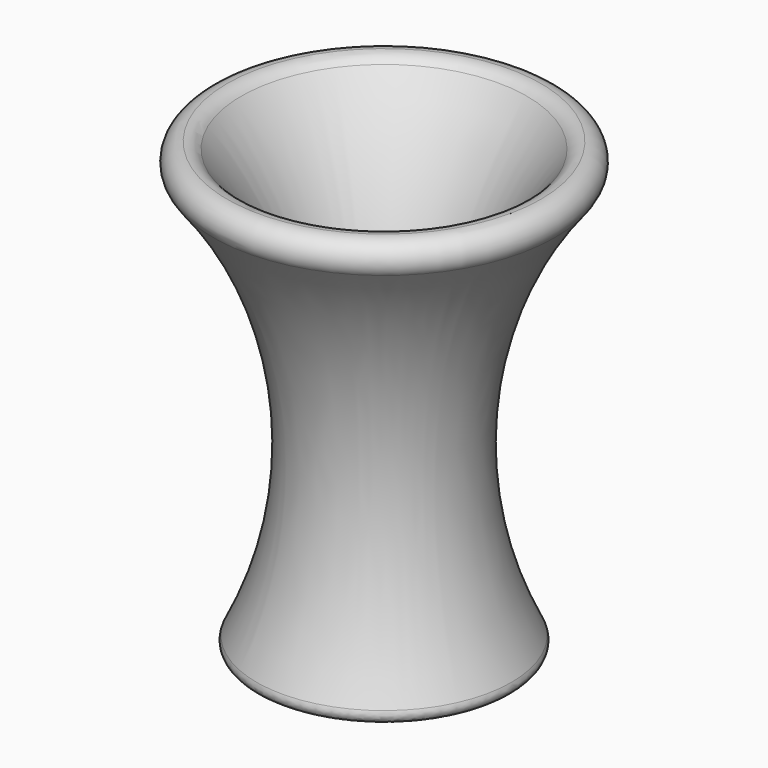
from build123d import *

# Parameters (mm, degrees)
F2_T = -5.08
F4_R = 2.54
F5_R = 1.27


# Not quite as in the source:
# - a fillet or chamfer that OpenCascade refuses, or shapes differently, is made with other operations: its cross-section is extruded or revolved along the edge and cut away or added


with BuildPart() as f1:
    # F0 (on Front) → F1 (revolve)
    with BuildSketch(Plane.XZ):
        with BuildLine():
            Line((67.6932582283, 49.1091830879), (39.7532582283, 49.1091830879))
            Line((39.7532582283, 49.1091830879), (39.7532582283, -14.3908169121))
            Line((39.7532582283, -14.3908169121), (58.8032582283, -14.3908169121))
            ThreePointArc((58.8032582283, -14.3908169121), (52.6399701012, 18.8443434257), (67.6932582283, 49.1091830879))
        make_face()
    revolve(axis=Axis((39.7532582283, 0, 17.3591830879), (0, 0, -1)))

    # F2
    f2_openings = [f1.faces().sort_by_distance(p)[0] for p in [
        (39.753258, 0, 49.109183),
    ]]
    offset(amount=F2_T, openings=f2_openings)

    # F3: fillet of radius 2.54 on 2 edges, made by hand

    # F3_s1 → F3_t2 (revolve, cut)
    with BuildSketch(Plane.XZ):
        with BuildLine():
            ThreePointArc((62.0020141866, 49.1091830879), (60.9074002922, 48.8612172112), (60.0265083615, 48.1657346014))
            ThreePointArc((60.0265083615, 48.1657346014), (60.413510259, 48.6394982972), (60.805452481, 49.1091830879))
            Line((60.805452481, 49.1091830879), (62.0020141866, 49.1091830879))
        make_face()
    revolve(axis=Axis((39.7532582283, 0, 49.1091830879), (0, 0, -1)), mode=Mode.SUBTRACT)

    # F3_s3 → F3_t4 (revolve, cut)
    with BuildSketch(Plane.XZ):
        with BuildLine():
            ThreePointArc((63.9775200117, 44.9726315745), (64.2940483099, 47.6637969824), (62.0020141866, 49.1091830879))
            Line((62.0020141866, 49.1091830879), (67.6932582283, 49.1091830879))
            ThreePointArc((67.6932582283, 49.1091830879), (65.7814432363, 47.0893652753), (63.9775200117, 44.9726315745))
        make_face()
    revolve(axis=Axis((39.7532582283, 0, 49.1091830879), (0, 0, -1)), mode=Mode.SUBTRACT)

    # F4
    f4_edges = [f1.edges().sort_by_distance(p)[0] for p in [
        (28.647756, 0, -9.310817),
    ]]
    fillet(f4_edges, radius=F4_R)

    # F5
    f5_edges = [f1.edges().sort_by_distance(p)[0] for p in [
        (20.703258, 0, -14.390817),
    ]]
    fillet(f5_edges, radius=F5_R)


solid = f1.part
